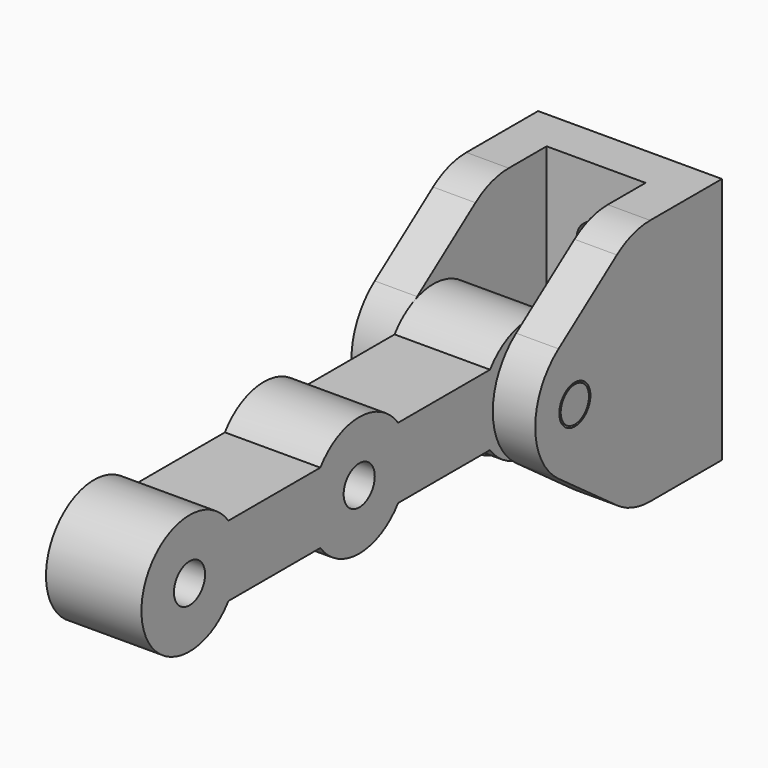
from build123d import *

# Parameters (mm, degrees)
F0_W     = 14
F0_H     = 35
F0_R     = 2.25
F0_R_2   = 2.75
F1_DEPTH = 6
F2_R     = 2.75
F2_W     = 6
F2_H     = 35
F3_DEPTH = 6
F4_R     = 2.75
F4_W     = 6
F4_H     = 35
F5_DEPTH = 6
F6_R     = 2.5
F7_DEPTH = 26
F8_R     = 2.75
F9_DEPTH = 13.5


with BuildPart() as f1:
    # F0 (on Front) → F1 (new body)
    with BuildSketch(Plane.XZ):
        with Locations((7, 17.5)):
            Rectangle(F0_W, F0_H)
        with Locations((7, 10)):
            Circle(F0_R, mode=Mode.SUBTRACT)
        with Locations((7, 25)):
            Circle(F0_R_2, mode=Mode.SUBTRACT)
    extrude(amount=F1_DEPTH)

    # F2 (on face) → F3 (join)
    with BuildSketch(Plane.YZ.offset(14)):
        with BuildLine():
            Line((-6, 0), (-6, 35))
            Line((-6, 35), (-12.6892046863, 35))
            ThreePointArc((-12.6892046863, 35), (-15.7820203249, 34.5097051177), (-18.5715576275, 33.0868982852))
            Line((-18.5715576275, 33.0868982852), (-28.8823529412, 25.5868982852))
            ThreePointArc((-28.8823529412, 25.5868982852), (-33, 17.5), (-28.8823529412, 9.4131017148))
            Line((-28.8823529412, 9.4131017148), (-18.5715576275, 1.9131017148))
            ThreePointArc((-18.5715576275, 1.9131017148), (-15.7820203249, 0.4902948823), (-12.6892046863, 0))
            Line((-12.6892046863, 0), (-6, 0))
        make_face()
        with Locations((-26, 17.5)):
            Circle(F2_R, mode=Mode.SUBTRACT)
        with Locations((-3, 17.5)):
            Rectangle(F2_W, F2_H)
    extrude(amount=F3_DEPTH)

    # F4 (on face) → F5 (join)
    with BuildSketch(Plane(origin=(0, 0, 0), x_dir=(0, -1, 0), z_dir=(-1, 0, 0))):
        with BuildLine():
            Line((12.6892046863, 35), (6, 35))
            Line((6, 35), (6, 0))
            Line((6, 0), (12.6892046863, 0))
            ThreePointArc((12.6892046863, 0), (15.7820203249, 0.4902948823), (18.5715576275, 1.9131017148))
            Line((18.5715576275, 1.9131017148), (28.8823529412, 9.4131017148))
            ThreePointArc((28.8823529412, 9.4131017148), (33, 17.5), (28.8823529412, 25.5868982852))
            Line((28.8823529412, 25.5868982852), (18.5715576275, 33.0868982852))
            ThreePointArc((18.5715576275, 33.0868982852), (15.7820203249, 34.5097051177), (12.6892046863, 35))
        make_face()
        with Locations((26, 17.5)):
            Circle(F4_R, mode=Mode.SUBTRACT)
        with Locations((3, 17.5)):
            Rectangle(F4_W, F4_H)
    extrude(amount=F5_DEPTH)


with BuildPart() as f7:
    # F6 (on face) → F7 (new body)
    with BuildSketch(Plane.YZ.offset(20)):
        with Locations((-26, 17.5)):
            Circle(F6_R)
    extrude(amount=-F7_DEPTH)


with BuildPart() as f9:
    # F8 (on face) → F9 (new body)
    with BuildSketch(Plane.YZ):
        with BuildLine():
            Line((-49.1261364576, 12.5), (-32.8738635424, 12.5))
            ThreePointArc((-32.8738635424, 12.5), (-17.5, 17.5), (-32.8738635424, 22.5))
            Line((-32.8738635424, 22.5), (-49.1261364576, 22.5))
            ThreePointArc((-49.1261364576, 22.5), (-56, 26), (-62.8738635424, 22.5))
            Line((-62.8738635424, 22.5), (-79.1261364576, 22.5))
            ThreePointArc((-79.1261364576, 22.5), (-94.5, 17.5), (-79.1261364576, 12.5))
            Line((-79.1261364576, 12.5), (-62.8738635424, 12.5))
            ThreePointArc((-62.8738635424, 12.5), (-56, 9), (-49.1261364576, 12.5))
        make_face()
        with Locations((-86, 17.5)):
            Circle(F8_R, mode=Mode.SUBTRACT)
        with Locations((-56, 17.5)):
            Circle(F8_R, mode=Mode.SUBTRACT)
        with Locations((-26, 17.5)):
            Circle(F8_R, mode=Mode.SUBTRACT)
    extrude(amount=F9_DEPTH)


solid = Compound([f1.part, f7.part, f9.part])
